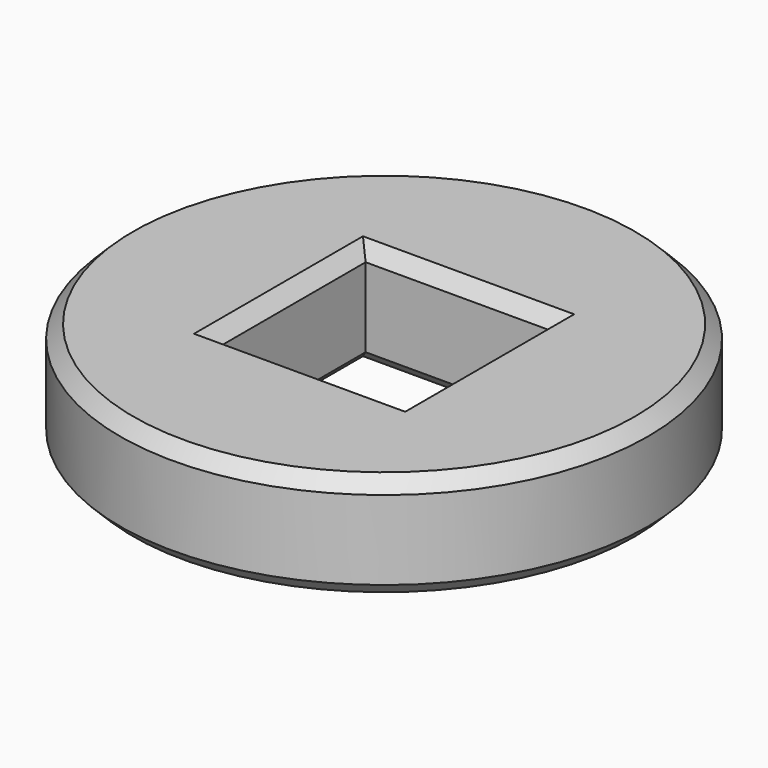
from build123d import *

# Parameters (mm, degrees)
F0_R     = 10
F0_W     = 7
F0_H     = 7
F1_DEPTH = 4
F2_SIZE  = 0.5
F3_SIZE  = 0.5


with BuildPart() as f1:
    # F0 (on Top) → F1 (new body)
    with BuildSketch(Plane.XY):
        Circle(F0_R)
        Rectangle(F0_W, F0_H, mode=Mode.SUBTRACT)
    extrude(amount=F1_DEPTH)

    # F2
    f2_edges = [f1.edges().sort_by_distance(p)[0] for p in [
        (-10, 0, 4),
        (-10, 0, 0),
        (-3.5, 0, 0),
        (-3.5, 0, 4),
    ]]
    chamfer(f2_edges, length=F2_SIZE)

    # F3
    f3_edges = [f1.edges().sort_by_distance(p)[0] for p in [
        (0, 3.5, 4),
        (3.5, 0, 4),
        (0, -3.5, 4),
        (0, -3.5, 0),
        (0, 3.5, 0),
        (3.5, 0, 0),
        (-3.75, -3.5, 0),
        (-3.75, 3.5, 0),
        (-3.75, -3.5, 4),
        (-3.75, 3.5, 4),
    ]]
    chamfer(f3_edges, length=F3_SIZE)


solid = f1.part
